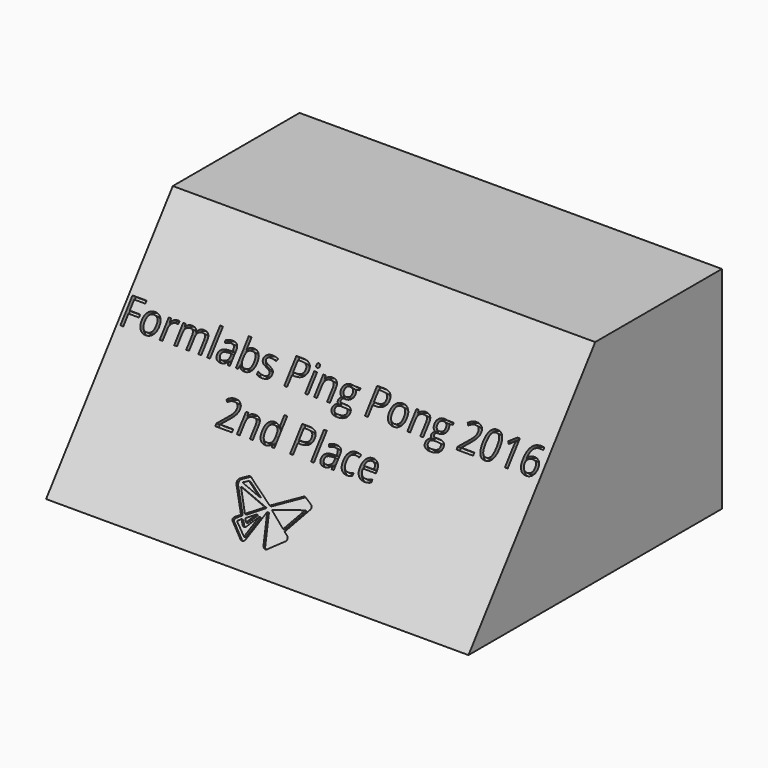
from build123d import *

# Parameters (mm, degrees)
F0_W         = 101.6
F0_H         = 76.2
F1_DEPTH     = 50.8
F3_DEPTH     = 101.601
F4_T         = -2.54
F5_TEXT_SIZE = 8.5353903059
F6_DEPTH     = 1.27
F8_DEPTH     = 0.635
F9_TEXT_SIZE = 4.2819676714
F10_DEPTH    = 1.27


# Not quite as in the source:
# - Text() gives the source's letters only with a copy of the font that has no kerning and outlines rounded to 1/6400 em; it was checked with that copy


with BuildPart() as f1:
    # F0 (on Top) → F1 (new body)
    with BuildSketch(Plane.XY):
        with Locations((16.9333308506, 38.1)):
            Rectangle(F0_W, F0_H)
    extrude(amount=F1_DEPTH)

    # F2 (on face) → F3 (cut, through all)
    with BuildSketch(Plane.YZ.offset(67.7333308506)):
        Polygon((0, 50.8), (0, 0), (38.1, 50.8), align=None)
    extrude(amount=-F3_DEPTH, mode=Mode.SUBTRACT)

    # F4
    f4_openings = [f1.faces().sort_by_distance(p)[0] for p in [
        (16.933331, 38.1, 0),
    ]]
    offset(amount=F4_T, openings=f4_openings)

    # F5 (on face) → F6 (cut)
    with BuildSketch(Plane(origin=(0, 0, 0), x_dir=(1, 0, 0), z_dir=(0, -0.8, 0.6))):
        with Locations((-33.878014423, 35.4853495955)):
            Text('Formlabs Ping Pong 2016', F5_TEXT_SIZE, font='Open Sans', text_align=(TextAlign.LEFT, TextAlign.BOTTOM))
        with Locations((-5.0457327007, 23.8772187796)):
            Text('2nd Place', F5_TEXT_SIZE, font='Open Sans', text_align=(TextAlign.LEFT, TextAlign.BOTTOM))
    extrude(amount=-F6_DEPTH, mode=Mode.SUBTRACT)

    # F7 (on face) → F8 (cut)
    with BuildSketch(Plane(origin=(0, 0, 0), x_dir=(1, 0, 0), z_dir=(0, -0.8, 0.6))):
        with BuildLine():
            Line((13.4837115183, 13.4272510186), (7.3560709134, 17.118493095))
            ThreePointArc((7.3560709134, 17.118493095), (6.9598628009, 17.3219317084), (6.5232547931, 17.2339454293))
            Line((6.5232547931, 17.2339454293), (5.0372248515, 16.3523033261))
            ThreePointArc((5.0372248515, 16.3523033261), (4.5941037589, 15.7553422177), (4.7088782303, 15.0208044797))
            Line((4.7088782303, 15.0208044797), (8.2500472502, 9.9444482787))
            Line((8.2500472502, 9.9444482787), (7.0838008274, 9.1308970741))
            ThreePointArc((7.0838008274, 9.1308970741), (6.8475814061, 8.6456949987), (7.1361442097, 8.1896772608))
            Line((7.1361442097, 8.1896772608), (10.2178193629, 5.5576669984))
            ThreePointArc((10.2178193629, 5.5576669984), (10.8682715637, 5.4446336831), (11.3433087245, 5.9031140991))
            Line((11.3433087245, 5.9031140991), (13.5008823127, 12.1355671436))
            Line((13.5008823127, 12.1355671436), (15.5845545232, 5.9314654209))
            ThreePointArc((15.5845545232, 5.9314654209), (15.9616371116, 5.4979932508), (16.5347233415, 5.4572308436))
            Line((16.5347233415, 5.4572308436), (19.7310019284, 8.081631735))
            ThreePointArc((19.7310019284, 8.081631735), (20.041796176, 8.6354321435), (19.7362490992, 9.1921447629))
            Line((19.7362490992, 9.1921447629), (18.8143051114, 9.7729407743))
            Line((18.8143051114, 9.7729407743), (22.2590983821, 15.2411368069))
            ThreePointArc((22.2590983821, 15.2411368069), (22.3842901343, 15.813418361), (22.0345240086, 16.2833575159))
            Line((22.0345240086, 16.2833575159), (20.3393120319, 17.2168835998))
            ThreePointArc((20.3393120319, 17.2168835998), (19.9693319663, 17.2853947372), (19.6317466821, 17.1192165172))
            Line((19.6317466821, 17.1192165172), (13.4837115183, 13.4272510186))
        make_face()
        with BuildLine():
            Line((10.2651705965, 8.0516058952), (12.2502879319, 10.7989438046))
            Line((12.2502879319, 10.7989438046), (10.7283759862, 6.2629207969))
            Line((10.7283759862, 6.2629207969), (7.9214246944, 8.5824187845))
            Line((7.9214246944, 8.5824187845), (8.7465365849, 9.2327181414))
            Line((8.7465365849, 9.2327181414), (9.4287740067, 8.2547133788))
            ThreePointArc((9.4287740067, 8.2547133788), (9.8085458541, 7.9949195314), (10.2651705965, 8.0516058952))
        make_face(mode=Mode.SUBTRACT)
        Polygon((9.4586731866, 9.6149612218), (11.4831300452, 11.0469274223), (9.9453385919, 8.9157661423), align=None, mode=Mode.SUBTRACT)
        Polygon((5.8720999334, 14.8942405851), (12.6240206882, 12.8366881981), (8.9787328616, 10.3465225548), align=None, mode=Mode.SUBTRACT)
        Polygon((5.7934536599, 15.7347135246), (7.0594344288, 16.4298992604), (10.5455731973, 14.3083883449), align=None, mode=Mode.SUBTRACT)
        Polygon((14.2554277554, 12.8213027492), (21.3006008416, 14.9052804336), (18.2668808848, 10.1485736668), align=None, mode=Mode.SUBTRACT)
    extrude(amount=-F8_DEPTH, mode=Mode.SUBTRACT)

    # F9 (on face) → F10 (cut)
    with BuildSketch(Plane.XZ.offset(-73.66)):
        with Locations((-14.5403649658, 11.9274128228)):
            Text('Designed & Printed by David Liu', F9_TEXT_SIZE, font='Open Sans', text_align=(TextAlign.LEFT, TextAlign.BOTTOM))
    extrude(amount=-F10_DEPTH, mode=Mode.SUBTRACT)


solid = f1.part
